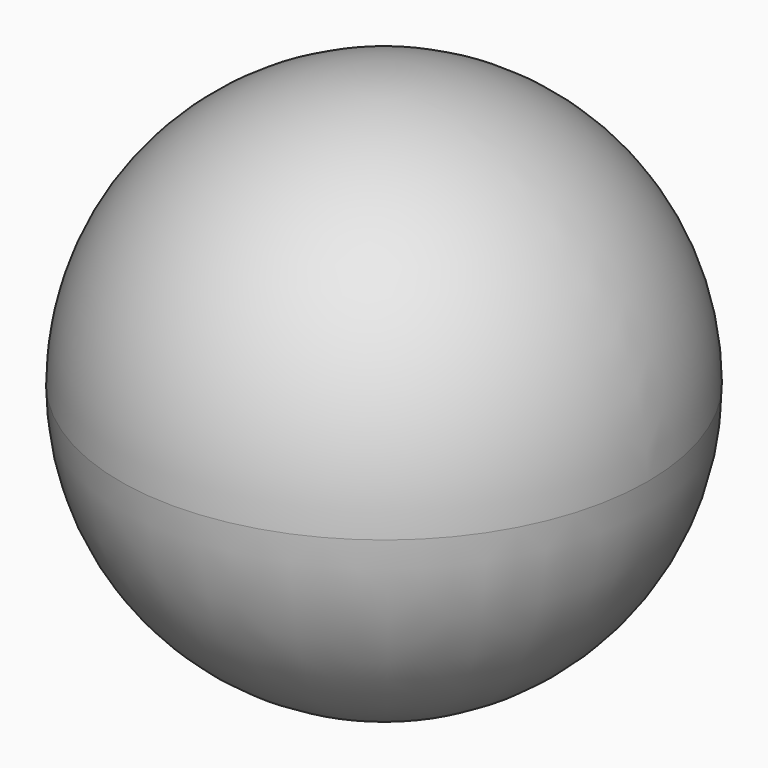
from build123d import *

# Parameters (mm, degrees)
F0_R     = 5
F1_DEPTH = 10
F2_R     = 5
F3_R     = 4.99999


# Not quite as in the source:
# - a fillet or chamfer is up to 0.001 mm smaller than in the source, because OpenCascade refuses the exact size


with BuildPart() as f1:
    # F0 (on Top) → F1 (new body)
    with BuildSketch(Plane.XY):
        Circle(F0_R)
    extrude(amount=F1_DEPTH)

    # F2
    f2_edges = [f1.edges().sort_by_distance(p)[0] for p in [
        (-5, 0, 10),
    ]]
    fillet(f2_edges, radius=F2_R)

    # F3 (radius 5 in the source; OpenCascade refuses exactly that, so slightly less here)
    f3_edges = [f1.edges().sort_by_distance(p)[0] for p in [
        (-5, 0, 0),
    ]]
    fillet(f3_edges, radius=F3_R)


solid = f1.part
